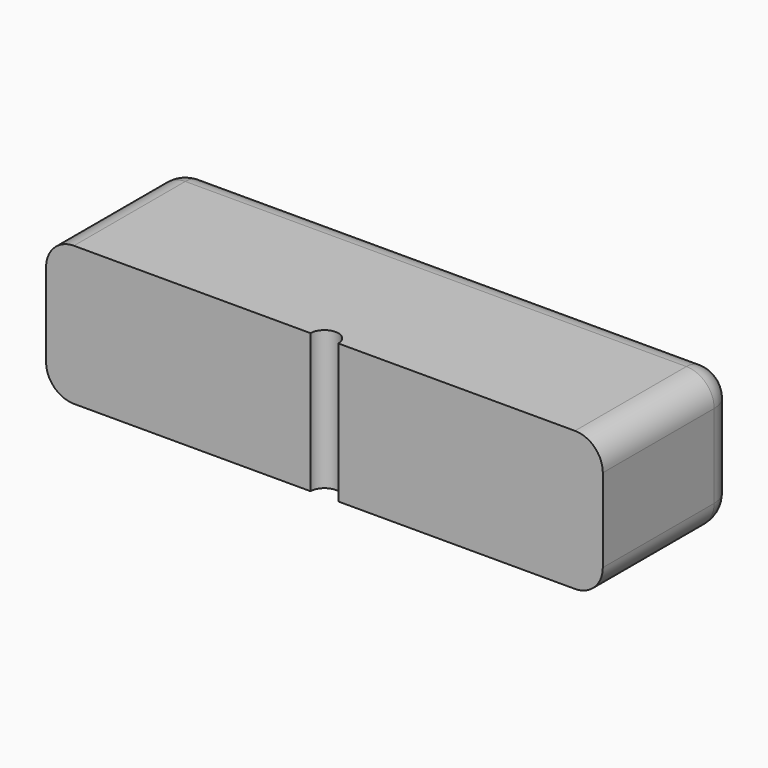
from build123d import *

# Parameters (mm, degrees)
F1_DEPTH     = 10
F2_R         = 2
F3_T1_DEPTH  = 15
F3_T3_DEPTH  = 6
F3_T5_DEPTH  = 36
F3_S9_W      = 2
F3_S9_H      = 2
F3_T10_DEPTH = 2
F3_S15_W     = 2
F3_S15_H     = 2
F3_T16_DEPTH = 2
F3_S21_W     = 2
F3_S21_H     = 2
F3_T22_DEPTH = 2
F3_S27_W     = 2
F3_S27_H     = 2
F3_T28_DEPTH = 2


# Not quite as in the source:
# - a fillet or chamfer that OpenCascade refuses, or shapes differently, is made with other operations: its cross-section is extruded or revolved along the edge and cut away or added


with BuildPart() as f1:
    # F0 (on Top) → F1 (new body)
    with BuildSketch(Plane.XY):
        with BuildLine():
            Line((40, 17.25), (0, 17.25))
            Line((0, 17.25), (0, 5.25))
            Line((0, 5.25), (19, 5.25))
            ThreePointArc((19, 5.25), (20, 6.25), (21, 5.25))
            Line((21, 5.25), (40, 5.25))
            Line((40, 5.25), (40, 17.25))
        make_face()
    extrude(amount=F1_DEPTH)

    # F2
    f2_edges = [f1.edges().sort_by_distance(p)[0] for p in [
        (0, 11.25, 0),
        (0, 11.25, 10),
        (0, 17.25, 5),
    ]]
    fillet(f2_edges, radius=F2_R)

    # F3: fillet of radius 2 on 5 edges, made by hand

    # F3_s2 → F3_t1 (cut)
    with BuildSketch(Plane.XZ.offset(-15.25)):
        with BuildLine():
            ThreePointArc((38, 0), (39.4142135624, 0.5857864376), (40, 2))
            Line((40, 2), (40, 0))
            Line((40, 0), (38, 0))
        make_face()
        with BuildLine():
            ThreePointArc((40, 8), (39.4142135624, 9.4142135624), (38, 10))
            Line((38, 10), (40, 10))
            Line((40, 10), (40, 8))
        make_face()
    extrude(amount=F3_T1_DEPTH, mode=Mode.SUBTRACT)

    # F3_s4 → F3_t3 (cut)
    with BuildSketch(Plane.XY.offset(2)):
        with BuildLine():
            ThreePointArc((38, 17.25), (39.4142135624, 16.6642135624), (40, 15.25))
            Line((40, 15.25), (40, 17.25))
            Line((40, 17.25), (38, 17.25))
        make_face()
    extrude(amount=F3_T3_DEPTH, mode=Mode.SUBTRACT)

    # F3_s6 → F3_t5 (cut)
    with BuildSketch(Plane.YZ.offset(2)):
        with BuildLine():
            ThreePointArc((17.25, 2), (16.6642135624, 0.5857864376), (15.25, 0))
            Line((15.25, 0), (17.25, 0))
            Line((17.25, 0), (17.25, 2))
        make_face()
        with BuildLine():
            ThreePointArc((17.25, 8), (16.6642135624, 9.4142135624), (15.25, 10))
            Line((15.25, 10), (17.25, 10))
            Line((17.25, 10), (17.25, 8))
        make_face()
    extrude(amount=F3_T5_DEPTH, mode=Mode.SUBTRACT)


with BuildPart() as f3_tool8:
    # F3_s9 → F3_t10 (new body)
    with BuildSketch(Plane.XZ.offset(-15.25)):
        with Locations((1, 9)):
            Rectangle(F3_S9_W, F3_S9_H)
    extrude(amount=-F3_T10_DEPTH)

    # F3_s11 → F3_t12 (revolve, cut)
    with BuildSketch(Plane(origin=(2, 15.25, 8), x_dir=(0.7071067812, 0, -0.7071067812), z_dir=(0.7071067812, 0, 0.7071067812))):
        with BuildLine():
            ThreePointArc((0, -2), (2, 0), (0, 2))
            Line((0, 2), (0, -2))
        make_face()
    revolve(axis=Axis((2, 15.25, 8), (0, 1, 0)), mode=Mode.SUBTRACT)


with BuildPart() as f1_1:
    add(f1.part)

    # F3_t7: cut F3_tool8
    add(f3_tool8.part, mode=Mode.SUBTRACT)


with BuildPart() as f3_tool14:
    # F3_s15 → F3_t16 (new body)
    with BuildSketch(Plane.XZ.offset(-15.25)):
        with Locations((1, 1)):
            Rectangle(F3_S15_W, F3_S15_H)
    extrude(amount=-F3_T16_DEPTH)

    # F3_s17 → F3_t18 (revolve, cut)
    with BuildSketch(Plane(origin=(2, 15.25, 2), x_dir=(0.7071067812, 0, 0.7071067812), z_dir=(-0.7071067812, 0, 0.7071067812))):
        with BuildLine():
            ThreePointArc((0, -2), (2, 0), (0, 2))
            Line((0, 2), (0, -2))
        make_face()
    revolve(axis=Axis((2, 15.25, 2), (0, 1, 0)), mode=Mode.SUBTRACT)


with BuildPart() as f1_2:
    add(f1_1.part)

    # F3_t13: cut F3_tool14
    add(f3_tool14.part, mode=Mode.SUBTRACT)


with BuildPart() as f3_tool20:
    # F3_s21 → F3_t22 (new body)
    with BuildSketch(Plane.XZ.offset(-15.25)):
        with Locations((39, 1)):
            Rectangle(F3_S21_W, F3_S21_H)
    extrude(amount=-F3_T22_DEPTH)

    # F3_s23 → F3_t24 (revolve, cut)
    with BuildSketch(Plane(origin=(38, 15.25, 2), x_dir=(-0.7071067812, 0, 0.7071067812), z_dir=(-0.7071067812, 0, -0.7071067812))):
        with BuildLine():
            ThreePointArc((0, -2), (2, 0), (0, 2))
            Line((0, 2), (0, -2))
        make_face()
    revolve(axis=Axis((38, 15.25, 2), (0, 1, 0)), mode=Mode.SUBTRACT)


with BuildPart() as f1_3:
    add(f1_2.part)

    # F3_t19: cut F3_tool20
    add(f3_tool20.part, mode=Mode.SUBTRACT)


with BuildPart() as f3_tool26:
    # F3_s27 → F3_t28 (new body)
    with BuildSketch(Plane.XZ.offset(-15.25)):
        with Locations((39, 9)):
            Rectangle(F3_S27_W, F3_S27_H)
    extrude(amount=-F3_T28_DEPTH)

    # F3_s29 → F3_t30 (revolve, cut)
    with BuildSketch(Plane(origin=(38, 15.25, 8), x_dir=(-0.7071067812, 0, -0.7071067812), z_dir=(0.7071067812, 0, -0.7071067812))):
        with BuildLine():
            ThreePointArc((0, -2), (2, 0), (0, 2))
            Line((0, 2), (0, -2))
        make_face()
    revolve(axis=Axis((38, 15.25, 8), (0, 1, 0)), mode=Mode.SUBTRACT)


with BuildPart() as f1_4:
    add(f1_3.part)

    # F3_t25: cut F3_tool26
    add(f3_tool26.part, mode=Mode.SUBTRACT)


solid = f1_4.part
